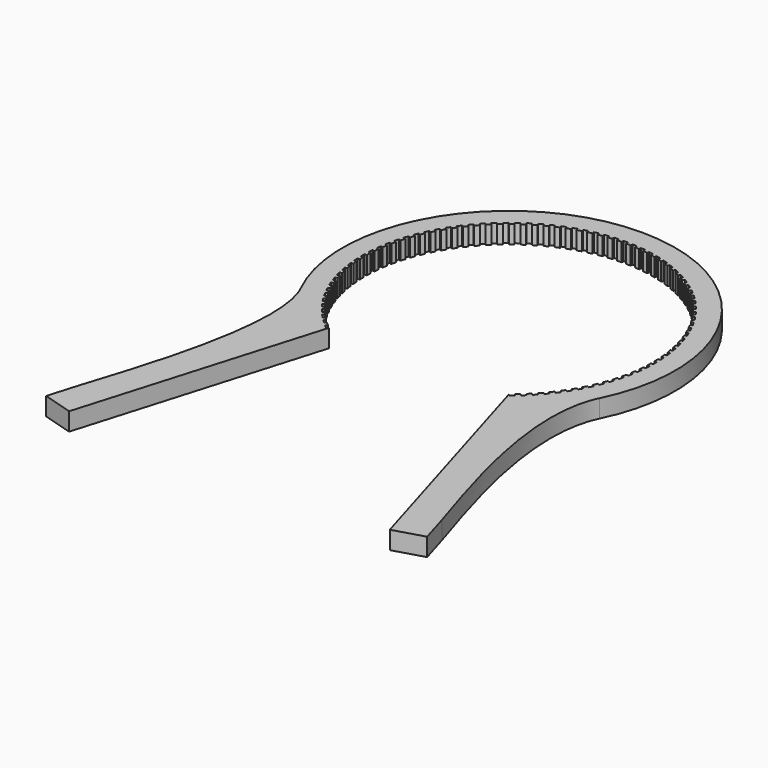
from build123d import *

# Parameters (mm, degrees)
F2_DEPTH         = 4
F4_DEPTH         = 4.0010001
F4_COPIES_COUNT  = 40
F4_COPIES_ANGLE  = 140.4
F4_COPIES1_COUNT = 40
F4_COPIES1_ANGLE = 140.4


# Not quite as in the source:
# - a pattern or mirror of a feature is missing from the dataset's text; its kind, count and spacing are read off the source's solid


with BuildPart() as f2:
    # F1 (on Top) → F2 (new body)
    with BuildSketch(Plane.XY):
        with BuildLine():
            add(Edge.make_bspline(
                [(40.4120250091, -69.107856701), (37.94537046, -60.804950863), (26.6053403245, -29.7340166268), (33.1981293463, -16.3365910735)],
                knots=[0, 0, 0, 0, 53.2620574759, 53.2620574759, 53.2620574759, 53.2620574759], degree=3))
            ThreePointArc((33.1981293463, -16.3365910735), (0, 37), (-33.1981293463, -16.3365910735))
            add(Edge.make_bspline(
                [(-40.4120250091, -69.107856701), (-37.94537046, -60.804950863), (-26.6053403245, -29.7340166268), (-33.1981293463, -16.3365910735)],
                knots=[0, 0, 0, 0, 53.2620574759, 53.2620574759, 53.2620574759, 53.2620574759], degree=3))
            Line((-40.4120250091, -69.107856701), (-42.3731441263, -75.7091002245))
            Line((-42.3731441263, -75.7091002245), (-35.6629974994, -77.7025726335))
            Line((-35.6629974994, -77.7025726335), (-20, -24.9799919936))
            ThreePointArc((-20, -24.9799919936), (0, 32), (20, -24.9799919936))
            Line((20, -24.9799919936), (35.6629974994, -77.7025726335))
            Line((35.6629974994, -77.7025726335), (42.3731441263, -75.7091002245))
            Line((42.3731441263, -75.7091002245), (40.4120250091, -69.107856701))
        make_face()
    extrude(amount=F2_DEPTH)

    # F3 (on Top) → F4 (cut, through all)
    with BuildSketch(Plane.XY):
        with BuildLine():
            ThreePointArc((-0.5, 31.9960935116), (0, 32), (0.5, 31.9960935116))
            Line((0.5, 31.9960935116), (0.5, 32.5))
            Line((0.5, 32.5), (0, 32.5))
            Line((0, 32.5), (-0.5, 32.5))
            Line((-0.5, 32.5), (-0.5, 31.9960935116))
        make_face()
    f4 = extrude(amount=F4_DEPTH, mode=Mode.SUBTRACT)

    # F4_copies: F4 ×40 about axis
    f4_copies_axis = Axis((0, 0, 0), (0, 0, 1))
    for i in range(1, F4_COPIES_COUNT):
        add(f4.rotate(f4_copies_axis, i * F4_COPIES_ANGLE / (F4_COPIES_COUNT - 1)), mode=Mode.SUBTRACT)

    # F4_copies1: F4 ×40 about axis
    f4_copies1_axis = Axis((0, 0, 0), (0, 0, -1))
    for i in range(1, F4_COPIES1_COUNT):
        add(f4.rotate(f4_copies1_axis, i * F4_COPIES1_ANGLE / (F4_COPIES1_COUNT - 1)), mode=Mode.SUBTRACT)


solid = f2.part
